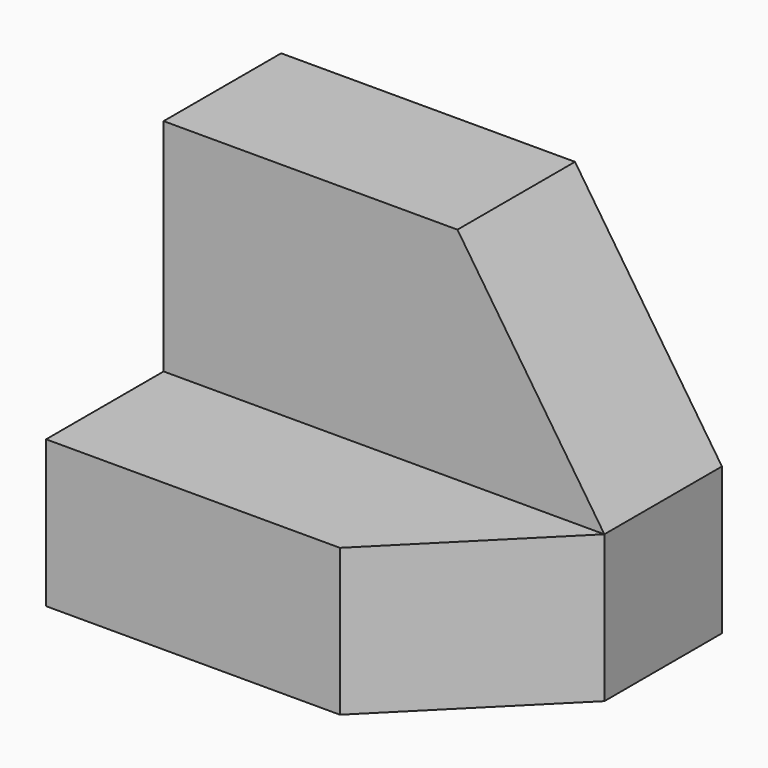
from build123d import *

# Parameters (mm, degrees)
F0_W     = 38.1
F0_H     = 31.75
F1_DEPTH = 25.4
F2_W     = 12.7
F2_H     = 19.05
F4_DEPTH = 12.7
F3_W     = 38.1
F3_H     = 19.05
F5_DEPTH = 12.7
F7_DEPTH = 12.701
F9_DEPTH = 12.701


# Not quite as in the source:
# - a feature names something its author has since deleted; it is built from what else it names


with BuildPart() as f1:
    # F0 (on Front) → F1 (new body)
    with BuildSketch(Plane.XZ):
        with Locations((19.05, 15.875)):
            Rectangle(F0_W, F0_H)
    extrude(amount=F1_DEPTH)

    # F2 (on face) → F4 (cut)
    with BuildSketch(Plane.YZ.offset(38.1)):
        with Locations((-19.05, 22.225)):
            Rectangle(F2_W, F2_H)
    extrude(amount=-F4_DEPTH, mode=Mode.SUBTRACT)

    # F3 (on face) → F5 (cut)
    with BuildSketch(Plane.XZ.offset(25.4)):
        with Locations((19.05, 22.225)):
            Rectangle(F3_W, F3_H)
    extrude(amount=-F5_DEPTH, mode=Mode.SUBTRACT)

    # F6 (on face) → F7 (cut, through all)
    with BuildSketch(Plane.XZ.offset(12.7)):
        Polygon((25.4, 31.75), (38.1, 12.7), (38.1, 31.75), align=None)
    extrude(amount=-F7_DEPTH, mode=Mode.SUBTRACT)

    # F8 (on face) → F9 (cut, through all)
    with BuildSketch(Plane.XY.offset(12.7)):
        Polygon((38.1, -25.4), (38.1, -12.7), (25.4, -25.4), align=None)
    extrude(amount=-F9_DEPTH, mode=Mode.SUBTRACT)


solid = f1.part
